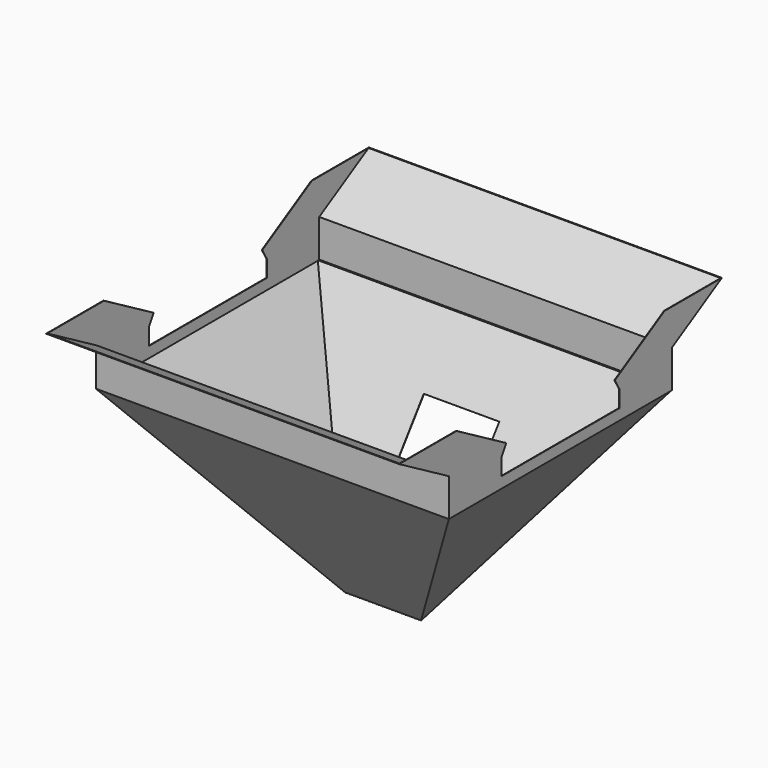
from build123d import *

# Parameters (mm, degrees)
F0_W        = 1870
F0_H        = 1469.5
F1_DEPTH    = 1011.3
F3_DEPTH    = 1870.001
F6_DEPTH    = 1469.501
F8_DEPTH    = 1870
F9_T        = 2.5
F9_T3_DEPTH = 1875
F10_W       = 400
F10_H       = 884.4916457885
F11_DEPTH   = 2.5


# Not quite as in the source:
# - a shell that OpenCascade refuses in one call is made with other operations: the cavity is built on its own and cut out


with BuildPart() as f1:
    # F0 (on Top) → F1 (new body)
    with BuildSketch(Plane.XY):
        with Locations((935, 734.75)):
            Rectangle(F0_W, F0_H)
    extrude(amount=-F1_DEPTH)

    # F2 (on face) → F3 (cut, through all)
    with BuildSketch(Plane.YZ.offset(1870)):
        Polygon((734.75, -1011.3), (0, 0), (0, -1011.3), align=None)
        Polygon((1469.5, 0), (734.75, -1011.3), (1469.5, -1011.3), align=None)
    extrude(amount=-F3_DEPTH, mode=Mode.SUBTRACT)

    # F5 (on face) → F6 (cut, through all)
    with BuildSketch(Plane(origin=(0, 0, 0), x_dir=(-1, 0, 0), z_dir=(0, 1, 0))):
        Polygon((0, -1011.0761593471), (0, 0), (-735, -1011.0761593471), (-1135, -1011.0761593471), (-1870, 0), (-1870, -1118.932723999), (0, -1118.932723999), align=None)
    extrude(amount=F6_DEPTH, mode=Mode.SUBTRACT)

    # F7 (on Right) → F8 (join)
    with BuildSketch(Plane.YZ):
        Polygon((0, 200), (0, 0), (739.4138846406, 0), (739.4138846406, 58.0384757729), (350, 58.0384757729), (350, 148.0384757729), (380, 200), (50.9103465619, 390), (-329.0896534381, 390), align=None)
        Polygon((739.4138846406, 58.0384757729), (739.4138846406, 0), (1478.8277692812, 0), (1478.8277692812, 200), (1807.9174227193, 390), (1427.9174227193, 390), (1098.8277692812, 200), (1128.8277692812, 148.0384757729), (1128.8277692812, 58.0384757729), align=None)
    extrude(amount=F8_DEPTH)

    # F9: shell of thickness 2.5, made by hand


with BuildPart() as f9_core1:
    # F9_t2: copy of F1
    add(f1.part)

    # the walls: a layer under each face that stays
    f9_faces = [f9_core1.faces().sort_by_distance(p)[0] for p in [
        (367.5, 734.75, -505.5380796735),
        (0, 27.0781925881, 65),
        (935, 367.2936853952, -505.5380796735),
        (935, 734.75, -1011.0761593471),
        (935, 1102.2063146048, -505.5380796735),
        (935, 0, 100),
        (935, 1474.1638846406, 0),
        (935, 1478.8277692812, 100),
        (935, 1643.3725960003, 295),
        (935, -164.544826719, 295),
        (1502.5, 734.75, -505.5380796735),
        (1870, 27.0781925881, 65),
    ]]
    thicken(f9_faces, amount=-F9_T, mode=Mode.SUBTRACT)

    # F9_s4 → F9_t3 (cut)
    with BuildSketch(Plane.YZ.offset(-2.5)):
        Polygon((1469.5202254482, -0.0396945991), (1467.4774551759, 1.4694599125), (1468.2261838709, 2.5), (1469.5, 2.5), align=None)
        Polygon((-0.0375, 199.9783493649), (2.5, 200), (2.5, 201.443375673), (1.25, 202.1650635095), align=None)
        Polygon((1478.8652692812, 199.9783493649), (1476.3277692812, 200), (1476.3277692812, 201.443375673), (1477.5777692812, 202.1650635095), align=None)
    extrude(amount=F9_T3_DEPTH, mode=Mode.SUBTRACT)


with BuildPart() as f1_1:
    add(f1.part)

    # what is left inside the walls is the cavity
    f9_cavity = [f9_core1.part.solids().sort_by_distance(p)[0] for p in [
        (1245.833333, 739.413885, 58.013476),
    ]]
    add(f9_cavity, mode=Mode.SUBTRACT)

    # F10 (on face) → F11 (cut)
    with BuildSketch(Plane(origin=(0, 961.8024604101, -698.7880527898), x_dir=(-1, 0, 0), z_dir=(0, 0.8090179296, -0.587783965))):
        with Locations((-935, 56.236940873)):
            Rectangle(F10_W, F10_H)
    extrude(amount=-F11_DEPTH, mode=Mode.SUBTRACT)


solid = f1_1.part
